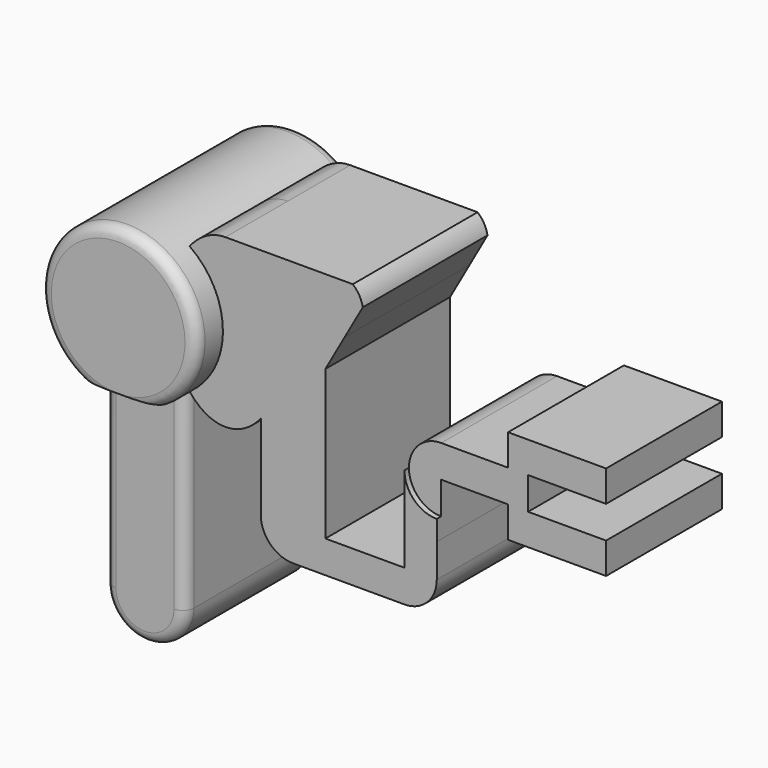
from build123d import *

# Parameters (mm, degrees)
F1_DEPTH = 2.5
F2_DEPTH = 1.75
F3_R     = 0.24999
F6_DEPTH = 1.75
F7_DEPTH = 1.75
F5_W     = 0.725
F5_H     = 0.725
F8_DEPTH = 1.75
F5_W_2   = 1.5000037169
F5_H_2   = 0.7249962804
F5_W_3   = 0.6
F5_H_3   = 0.6999998717
F5_H_4   = 0.6999961522
F9_DEPTH = 1.625


# Not quite as in the source:
# - a fillet or chamfer is up to 0.001 mm smaller than in the source, because OpenCascade refuses the exact size
# - ends of sketch curves that miss each other by under 0.0002 mm in the source are joined


with BuildPart() as f1:
    # F0 (on Front) → F1 (new body, symmetric)
    with BuildSketch(Plane.XZ):
        with BuildLine():
            Line((-0.9013878189, -1.5), (0.9013878189, -1.5))
            ThreePointArc((0.9013878189, -1.5), (0, 1.75), (-0.9013878189, -1.5))
        make_face()
    extrude(amount=F1_DEPTH, both=True)

    # F0 (on Front) → F2 (join, symmetric)
    with BuildSketch(Plane.XZ):
        with BuildLine():
            Line((0.9013878189, -5.8486121811), (0.9013878189, -1.5))
            Line((0.9013878189, -1.5), (-0.9013878189, -1.5))
            Line((-0.9013878189, -1.5), (-0.9013878189, -5.8486121811))
            ThreePointArc((-0.9013878189, -5.8486121811), (0, -6.75), (0.9013878189, -5.8486121811))
        make_face()
    extrude(amount=F2_DEPTH, both=True)

    # F3 (radius 0.25 in the source; OpenCascade refuses exactly that, so slightly less here)
    f3_edges = [f1.edges().sort_by_distance(p)[0] for p in [
        (-0.901388, -1.75, -3.674306),
        (0, -2.5, 1.75),
        (0, 2.5, 1.75),
    ]]
    fillet(f3_edges, radius=F3_R)


with BuildPart() as f6:
    # F5 (on Front) → F6 (new body, symmetric)
    with BuildSketch(Plane.XZ):
        with BuildLine():
            ThreePointArc((1.0024869547, 1.4344057675), (1.75, 0), (1.0024869547, -1.4344057675))
            add(Edge.make_bspline(
                [(1.0024869563, -1.4344057663), (1.7969250862, -2.4375739072), (2.6000000016, -1.4500000013)],
                knots=[5.5834557893, 5.5834557893, 5.5834557893, 6.9698995825, 6.9698995825, 6.9698995825], degree=2, weights=[1, 0.7691911586, 1]))
            add(Edge.make_bspline(
                [(2.6000000016, -1.4500000013), (5.303822052, 1.8750000109), (1.8075004381, 1.875)],
                knots=[0.6867142753, 0.6867142753, 0.6867142753, 3.1415926557, 3.1415926557, 3.1415926557], degree=2, weights=[1, 0.3366501631, 1]))
            add(Edge.make_bspline(
                [(1.8075004381, 1.875), (1.3514063883, 1.8749999986), (1.0024869563, 1.4344057663)],
                knots=[3.1415926557, 3.1415926557, 3.1415926557, 3.8413221714, 3.8413221714, 3.8413221714], degree=2, weights=[1, 0.9394190785, 1]))
        make_face()
    extrude(amount=F6_DEPTH, both=True)

    # F5 (on Front) → F7 (join, symmetric)
    with BuildSketch(Plane.XZ):
        with BuildLine():
            add(Edge.make_bspline(
                [(2.6000000016, -1.4500000013), (5.303822052, 1.8750000109), (1.8075004381, 1.875)],
                knots=[0.6867142753, 0.6867142753, 0.6867142753, 3.1415926557, 3.1415926557, 3.1415926557], degree=2, weights=[1, 0.3366501631, 1]))
            Line((2.6, -1.45), (2.6, -3.35))
            Line((2.6, -3.35), (4.05, -3.35))
            Line((4.05, -3.35), (4.05, 0))
            Line((4.05, 0), (4.4820705548, 0.7678400066))
            ThreePointArc((4.4820705548, 0.7678400066), (3.6888877758, 1.0468947244), (3.8346688069, 1.875))
            Line((3.8346688069, 1.875), (1.8075004381, 1.875))
        make_face()
        with BuildLine():
            Line((4.6653311931, 1.875), (3.8346688069, 1.875))
            ThreePointArc((3.8346688069, 1.875), (3.6888877758, 1.0468947244), (4.4820705548, 0.7678400066))
            Line((4.4820705548, 0.7678400066), (4.8894271065, 1.4917603336))
            ThreePointArc((4.8894271065, 1.4917603336), (4.8111122242, 1.7031052756), (4.6653311931, 1.875))
        make_face()
    extrude(amount=F7_DEPTH, both=True)

    # F5 (on Front) → F8 (join, symmetric)
    with BuildSketch(Plane.XZ):
        with BuildLine():
            Line((4.05, -3.35), (2.6, -3.35))
            ThreePointArc((2.6, -3.35), (2.8123475836, -3.8626524164), (3.325, -4.075))
            ThreePointArc((3.325, -4.075), (3.8376524164, -3.8626524164), (4.05, -3.35))
        make_face()
        with BuildLine():
            Line((5.1000000026, -3.35), (4.05, -3.35))
            ThreePointArc((4.05, -3.35), (3.8376524164, -3.8626524164), (3.325, -4.075))
            Line((3.325, -4.075), (5.1000000026, -4.075))
            Line((5.1000000026, -4.075), (5.1000000026, -3.35))
        make_face()
        with Locations((5.4625000026, -3.7125)):
            Rectangle(F5_W, F5_H)
        with BuildLine():
            Line((5.8250000026, -2.625), (5.8250000026, -3.35))
            Line((5.8250000026, -3.35), (5.8250000026, -4.075))
            ThreePointArc((5.8250000026, -4.075), (6.337652419, -3.8626524164), (6.5500000026, -3.35))
            ThreePointArc((6.5500000026, -3.35), (6.337652419, -2.8373475836), (5.8250000026, -2.625))
        make_face()
        with BuildLine():
            Line((5.8250000026, -2.5999961522), (5.8250000026, -2.625))
            ThreePointArc((5.8250000026, -2.625), (6.337652419, -2.8373475836), (6.5500000026, -3.35))
            Line((6.5500000026, -3.35), (6.5499962831, -2.5999961522))
            Line((6.5499962831, -2.5999961522), (5.8250000026, -2.5999961522))
        make_face()
        with BuildLine():
            Line((5.8250000026, -1.4249961522), (5.8250000026, -2.5999961522))
            Line((5.8250000026, -2.5999961522), (6.5499962831, -2.5999961522))
            Line((6.5499962831, -2.5999961522), (6.5499962831, -2.1499924326))
            ThreePointArc((6.5499962831, -2.1499924326), (6.0373464968, -1.9376459384), (5.8250000026, -1.4249961522))
        make_face()
    extrude(amount=F8_DEPTH, both=True)

    # F5 (on Front) → F9 (join, symmetric)
    with BuildSketch(Plane.XZ):
        with BuildLine():
            ThreePointArc((6.5499962831, -0.6999998717), (6.0373464968, -0.9123463659), (5.8250000026, -1.4249961522))
            ThreePointArc((5.8250000026, -1.4249961522), (6.0373464968, -1.9376459384), (6.5499962831, -2.1499924326))
            Line((6.5499962831, -2.1499924326), (6.5499962831, -1.4249961522))
            Line((6.5499962831, -1.4249961522), (6.5499962831, -0.6999998717))
        make_face()
        with Locations((7.2999981415, -1.0624980119)):
            Rectangle(F5_W_2, F5_H_2)
        Polygon((8.05, 0), (8.05, -0.6999998717), (8.05, -1.4249961522), (8.05, -2.1249961522), (9.65, -2.1249961522), (9.65, -1.425), (8.5, -1.425), (8.5, -0.6999998717), (9.65, -0.6999998717), (9.65, 0), align=None)
        with Locations((9.95, -0.3499999359)):
            Rectangle(F5_W_3, F5_H_3)
        with Locations((9.95, -1.7749980761)):
            Rectangle(F5_W_3, F5_H_4)
    extrude(amount=F9_DEPTH, both=True)


solid = Compound([f1.part, f6.part])
